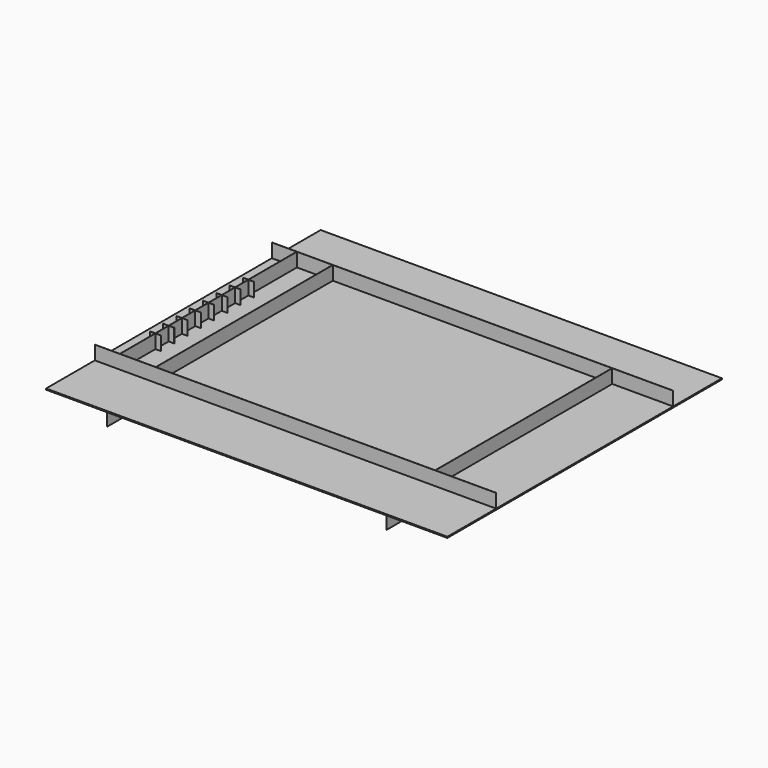
from build123d import *

# Parameters (mm, degrees)
F0_W     = 725
F0_H     = 620
F1_DEPTH = 2
F2_W     = 0.25
F2_H     = 110
F3_DEPTH = 25
F4_DEPTH = 25
F2_W_2   = 110
F2_H_2   = 0.2
F2_W_3   = 0.2
F2_H_3   = 399.6
F5_DEPTH = 25
F2_W_4   = 64.7
F6_DEPTH = 25
F2_W_5   = 45.1
F7_DEPTH = 25
F2_H_4   = 49.5626640439
F8_DEPTH = 25
F2_H_5   = 109.4
F2_W_6   = 9.8
F2_H_6   = 30.4373359561
F2_W_7   = 10
F2_H_7   = 29.8
F9_DEPTH = 25


# Not quite as in the source:
# - a feature names something its author has since deleted; it is built from what else it names


with BuildPart() as f1:
    # F0 (on Top) → F1 (new body)
    with BuildSketch(Plane.XY):
        with Locations((362.5, 310)):
            Rectangle(F0_W, F0_H)
    extrude(amount=F1_DEPTH)

    # F2 (on face) → F3 (join)
    with BuildSketch(Plane.XY.offset(2)):
        with Locations((614.875, 565)):
            Rectangle(F2_W, F2_H)
        with Locations((110.125, 565)):
            Rectangle(F2_W, F2_H)
        Polygon((110.2, 110), (110, 110), (110, 0), (110.25, 0), (110.25, 110), align=None)
        Polygon((615, 110), (614.8, 110), (614.75, 110), (614.75, 0), (615, 0), align=None)
    extrude(amount=-F3_DEPTH)

    # F2 (on face) → F4 (join)
    with BuildSketch(Plane.XY.offset(2)):
        Polygon((110, 510), (0, 510), (0, 509.8), (45.1, 509.8), (45.3, 509.8), (110, 509.8), align=None)
        Polygon((614.75, 510), (110.25, 510), (110.25, 509.8), (614.8, 509.8), (615, 509.8), (615, 510), align=None)
    extrude(amount=F4_DEPTH)

    # F2 (on face) → F5 (join)
    with BuildSketch(Plane.XY.offset(2)):
        with Locations((670, 509.9)):
            Rectangle(F2_W_2, F2_H_2)
        with Locations((614.9, 310)):
            Rectangle(F2_W_3, F2_H_3)
    extrude(amount=F5_DEPTH)

    # F2 (on face) → F6 (join)
    with BuildSketch(Plane.XY.offset(2)):
        with Locations((670, 110.1)):
            Rectangle(F2_W_2, F2_H_2)
        Polygon((614.8, 110.2), (110.2, 110.2), (110.2, 110), (110.25, 110), (614.75, 110), (614.8, 110), align=None)
        with Locations((614.9, 110.1)):
            Rectangle(F2_W_3, F2_H_2)
        with Locations((77.65, 110.1)):
            Rectangle(F2_W_4, F2_H_2)
        with Locations((110.1, 110.1)):
            Rectangle(F2_W_3, F2_H_2)
    extrude(amount=F6_DEPTH)

    # F2 (on face) → F7 (join)
    with BuildSketch(Plane.XY.offset(2)):
        with Locations((22.55, 110.1)):
            Rectangle(F2_W_5, F2_H_2)
    extrude(amount=F7_DEPTH)

    # F2 (on face) → F8 (join)
    with BuildSketch(Plane.XY.offset(2)):
        with Locations((45.2, 165.418667978)):
            Rectangle(F2_W_3, F2_H_4)
    extrude(amount=F8_DEPTH)

    # F2 (on face) → F9 (join)
    with BuildSketch(Plane.XY.offset(2)):
        Polygon((110.25, 510), (110, 510), (110, 509.8), (110.2, 509.8), (110.25, 509.8), align=None)
        with Locations((110.1, 310)):
            Rectangle(F2_W_3, F2_H_3)
        with Locations((45.2, 455.1)):
            Rectangle(F2_W_3, F2_H_5)
        with Locations((45.2, 400.3)):
            Rectangle(F2_W_3, F2_H_2)
        with Locations((40.2, 400.3)):
            Rectangle(F2_W_6, F2_H_2)
        with Locations((45.2, 125.418667978)):
            Rectangle(F2_W_3, F2_H_6)
        with Locations((45.2, 110.1)):
            Rectangle(F2_W_3, F2_H_2)
        with Locations((50.3, 400.3)):
            Rectangle(F2_W_7, F2_H_2)
        with Locations((45.2, 385.3)):
            Rectangle(F2_W_3, F2_H_7)
        with Locations((45.2, 165.418667978)):
            Rectangle(F2_W_3, F2_H_4)
        with Locations((45.2, 370.3)):
            Rectangle(F2_W_3, F2_H_2)
        with Locations((40.2, 370.3)):
            Rectangle(F2_W_6, F2_H_2)
        with Locations((40.2, 190.3)):
            Rectangle(F2_W_6, F2_H_2)
        with Locations((45.2, 190.3)):
            Rectangle(F2_W_3, F2_H_2)
        with Locations((50.3, 370.3)):
            Rectangle(F2_W_7, F2_H_2)
        with Locations((50.3, 190.3)):
            Rectangle(F2_W_7, F2_H_2)
        with Locations((45.2, 355.3)):
            Rectangle(F2_W_3, F2_H_7)
        with Locations((45.2, 205.3)):
            Rectangle(F2_W_3, F2_H_7)
        with Locations((45.2, 340.3)):
            Rectangle(F2_W_3, F2_H_2)
        with Locations((40.2, 340.3)):
            Rectangle(F2_W_6, F2_H_2)
        with Locations((40.2, 220.3)):
            Rectangle(F2_W_6, F2_H_2)
        with Locations((45.2, 220.3)):
            Rectangle(F2_W_3, F2_H_2)
        with Locations((50.3, 340.3)):
            Rectangle(F2_W_7, F2_H_2)
        with Locations((50.3, 220.3)):
            Rectangle(F2_W_7, F2_H_2)
        with Locations((45.2, 325.3)):
            Rectangle(F2_W_3, F2_H_7)
        with Locations((45.2, 235.3)):
            Rectangle(F2_W_3, F2_H_7)
        with Locations((45.2, 310.3)):
            Rectangle(F2_W_3, F2_H_2)
        with Locations((40.2, 310.3)):
            Rectangle(F2_W_6, F2_H_2)
        with Locations((40.2, 250.3)):
            Rectangle(F2_W_6, F2_H_2)
        with Locations((45.2, 250.3)):
            Rectangle(F2_W_3, F2_H_2)
        with Locations((50.3, 310.3)):
            Rectangle(F2_W_7, F2_H_2)
        with Locations((50.3, 250.3)):
            Rectangle(F2_W_7, F2_H_2)
        with Locations((45.2, 295.3)):
            Rectangle(F2_W_3, F2_H_7)
        with Locations((45.2, 265.3)):
            Rectangle(F2_W_3, F2_H_7)
        with Locations((45.2, 280.3)):
            Rectangle(F2_W_3, F2_H_2)
        with Locations((40.2, 280.3)):
            Rectangle(F2_W_6, F2_H_2)
        with Locations((50.3, 280.3)):
            Rectangle(F2_W_7, F2_H_2)
    extrude(amount=F9_DEPTH)


solid = f1.part
